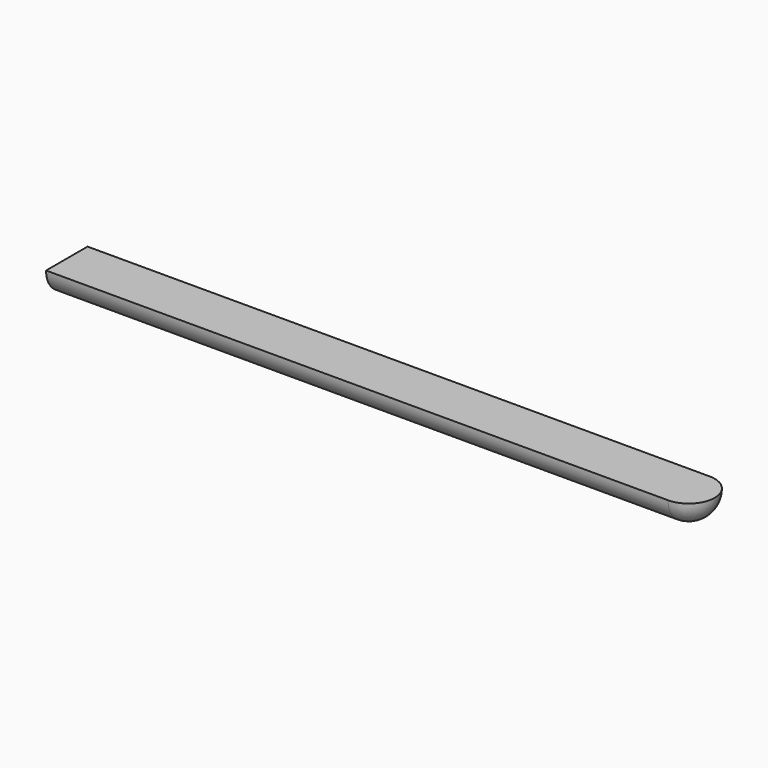
from build123d import *

# Parameters (mm, degrees)
F0_W     = 250
F0_H     = 10
F1_ANGLE = 180
F2_R     = 9.99999


# Not quite as in the source:
# - a fillet or chamfer is up to 0.001 mm smaller than in the source, because OpenCascade refuses the exact size


with BuildPart() as f1:
    # F0 (on Top) → F1 (revolve)
    with BuildSketch(Plane.XY):
        with Locations((0, -5)):
            Rectangle(F0_W, F0_H)
    revolve(axis=Axis((0, 0, 0), (1, 0, 0)), revolution_arc=F1_ANGLE)

    # F2 (radius 10 in the source; OpenCascade refuses exactly that, so slightly less here)
    f2_edges = [f1.edges().sort_by_distance(p)[0] for p in [
        (125, 0, -10),
    ]]
    fillet(f2_edges, radius=F2_R)


solid = f1.part
